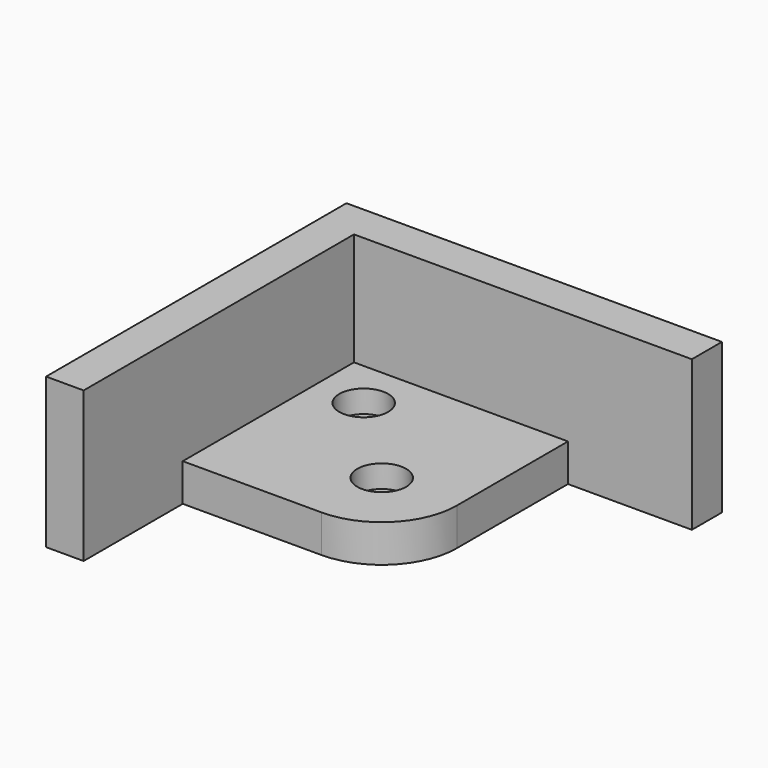
from build123d import *

# Parameters (mm, degrees)
F4_DEPTH       = 5
F5_DEPTH       = 20
F7_D           = 3.3
F7_CBORE_D     = 6.5
F7_CBORE_DEPTH = 3


# Not quite as in the source:
# - the program builds the solid bodies; features that only make, move or delete a surface that nothing else refers to are left out


with BuildPart() as f4:
    # F3 (on Top) → F4 (new body)
    with BuildSketch(Plane.XY):
        Polygon((-193.5, 232.5), (-193.5, 237.5), (-243.5, 237.5), (-243.5, 187.5), (-238.5, 187.5), (-238.5, 204), (-238.5, 232.5), (-210, 232.5), align=None)
        with BuildLine():
            Line((-210, 214), (-210, 232.5))
            Line((-210, 232.5), (-238.5, 232.5))
            Line((-238.5, 232.5), (-238.5, 204))
            Line((-238.5, 204), (-220, 204))
            ThreePointArc((-220, 204), (-227.0710678119, 221.0710678119), (-210, 214))
        make_face()
        with BuildLine():
            ThreePointArc((-220, 204), (-212.9289321881, 206.9289321881), (-210, 214))
            ThreePointArc((-210, 214), (-227.0710678119, 221.0710678119), (-220, 204))
        make_face()
    extrude(amount=F4_DEPTH)

    # F3 (on Top) → F5 (join)
    with BuildSketch(Plane.XY):
        Polygon((-193.5, 232.5), (-193.5, 237.5), (-243.5, 237.5), (-243.5, 187.5), (-238.5, 187.5), (-238.5, 204), (-238.5, 232.5), (-210, 232.5), align=None)
    extrude(amount=F5_DEPTH)

    # F7 (through all)
    with Locations(Plane.XY.offset(5)):
        with Locations((-232, 226), (-220, 214)):
            CounterBoreHole(F7_D / 2, F7_CBORE_D / 2, F7_CBORE_DEPTH)


solid = f4.part
